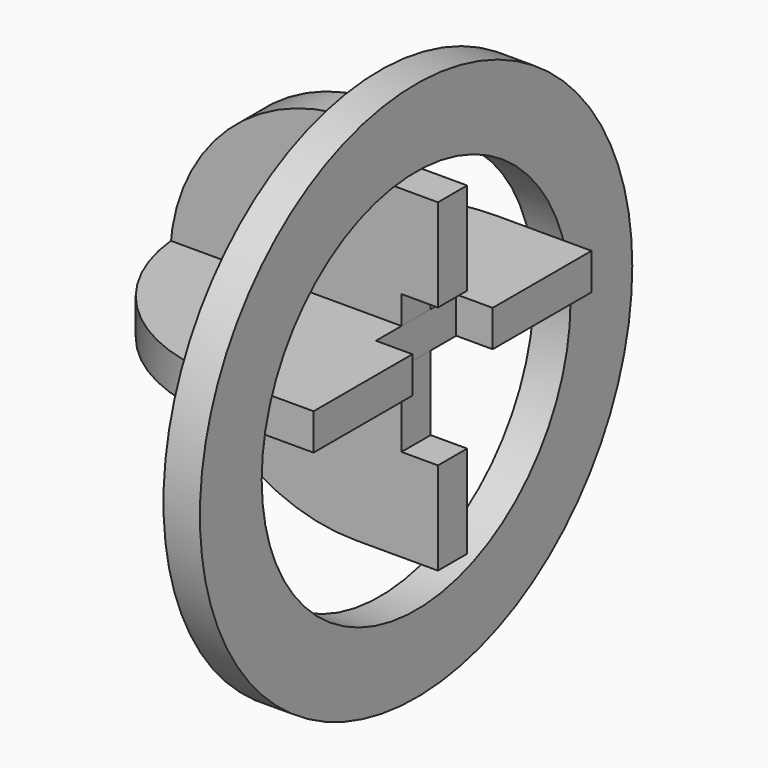
from build123d import *

# Parameters (mm, degrees)
F2_DEPTH  = 1.18
F4_DEPTH  = 1.18
F6_DEPTH  = 12.001
F7_R      = 17.5
F8_DEPTH  = 2.36
F9_R      = 12.5
F10_DEPTH = 15.001
F12_DEPTH = 14.501


with BuildPart() as f2:
    # F1 (on Top) → F2 (new body, symmetric)
    with BuildSketch(Plane.XY):
        with BuildLine():
            Line((2.36, 3.25), (2.36, 11.25))
            Line((2.36, 11.25), (0, 11.25))
            Line((0, 11.25), (-3.75, 11.25))
            ThreePointArc((-3.75, 11.25), (-15, 0), (-3.75, -11.25))
            Line((-3.75, -11.25), (0, -11.25))
            Line((0, -11.25), (2.36, -11.25))
            Line((2.36, -11.25), (2.36, -3.25))
            Line((2.36, -3.25), (0, -3.25))
            Line((0, -3.25), (0, 3.25))
            Line((0, 3.25), (2.36, 3.25))
        make_face()
    extrude(amount=F2_DEPTH, both=True)

    # F5 (on Top) → F6 (cut, through all)
    with BuildSketch(Plane.XY):
        Polygon((-6.64, -1.18), (-6.64, 0), (-6.64, 1.18), (-18.64, 1.18), (-18.64, -1.18), align=None)
    extrude(amount=-F6_DEPTH, mode=Mode.SUBTRACT)

    # F5 (on Top) → F12 (cut, through all)
    with BuildSketch(Plane.XY):
        Polygon((-6.64, -1.18), (-6.64, 0), (-6.64, 1.18), (-18.64, 1.18), (-18.64, -1.18), align=None)
    extrude(amount=F12_DEPTH, mode=Mode.SUBTRACT)


with BuildPart() as f4:
    # F3 (on Front) → F4 (new body, symmetric)
    with BuildSketch(Plane.XZ):
        with BuildLine():
            Line((2.36, 3), (2.36, 9))
            Line((2.36, 9), (0, 9))
            Line((0, 9), (-3, 9))
            Line((-3, 9), (-3, 12))
            ThreePointArc((-3, 12), (-15, 0), (-3, -12))
            Line((-3, -12), (0, -12))
            Line((0, -12), (2.36, -12))
            Line((2.36, -12), (2.36, -6))
            Line((2.36, -6), (0, -6))
            Line((0, -6), (0, 3))
            Line((0, 3), (2.36, 3))
        make_face()
    extrude(amount=F4_DEPTH, both=True)

    # F13: cut F2
    add(f2.part, mode=Mode.SUBTRACT)


with BuildPart() as f8:
    # F7 (on Right) → F8 (new body)
    with BuildSketch(Plane.YZ):
        Circle(F7_R)
    extrude(amount=-F8_DEPTH)

    # F9 (on Right) → F10 (cut, through all)
    with BuildSketch(Plane.YZ):
        Circle(F9_R)
    extrude(amount=-F10_DEPTH, mode=Mode.SUBTRACT)


with BuildPart() as f8_1:
    # F11: moved
    add(f8.part.moved(Location((0, 0, -3))))


solid = Compound([f2.part, f4.part, f8_1.part])
